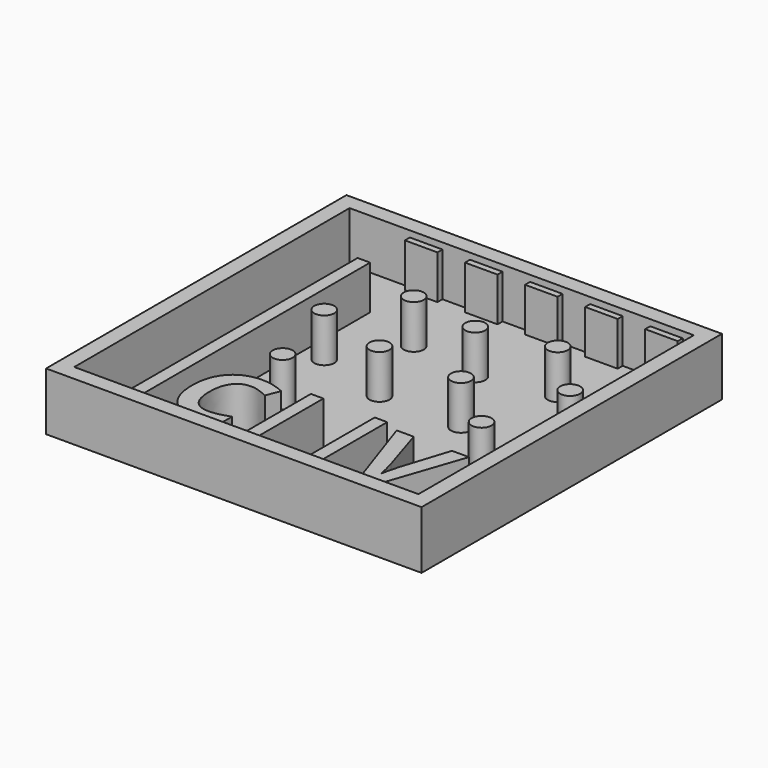
from build123d import *

# Parameters (mm, degrees)
F0_W         = 38.1
F0_H         = 38.1
F1_DEPTH     = 0.79375
F2_W         = 38.1
F2_H         = 38.1
F2_W_2       = 34.925
F2_H_2       = 34.925
F3_DEPTH     = 5.08
F4_R         = 1.27
F5_DEPTH     = 0.396875
F4_W         = 1.27
F4_H         = 29.591
F4_W_2       = 3.302
F4_H_2       = 0.635
F4_TEXT_SIZE = 11.2888888889
F4_R_2       = 1.016
F4_W_3       = 5.207
F4_H_3       = 0.508
F6_DEPTH     = 4.445


# Not quite as in the source:
# - a feature names something its author has since deleted; it is built from what else it names
# - Text() gives the source's letters only with a copy of the font that has no kerning and outlines rounded to 1/6400 em; it was checked with that copy


with BuildPart() as f1:
    # F0 (on Top) → F1 (new body)
    with BuildSketch(Plane.XY):
        with Locations((0, 3.0672513019)):
            Rectangle(F0_W, F0_H)
    extrude(amount=F1_DEPTH)

    # F2 (on face) → F3 (join)
    with BuildSketch(Plane.XY.offset(0.79375)):
        with Locations((0, 3.0672513019)):
            Rectangle(F2_W, F2_H)
        with Locations((0, 3.0672513019)):
            Rectangle(F2_W_2, F2_H_2, mode=Mode.SUBTRACT)
    extrude(amount=F3_DEPTH)

    # F4 (on face) → F5 (cut)
    with BuildSketch(Plane.XY.offset(0.79375)):
        with Locations((-14.9225, -11.5426807876)):
            Circle(F4_R)
        with Locations((3.175, -11.2202486981)):
            Circle(F4_R)
    extrude(amount=-F5_DEPTH, mode=Mode.SUBTRACT)

    # F4 (on face) → F6 (join)
    with BuildSketch(Plane.XY.offset(0.79375)):
        with Locations((-11.7475, 0.4002513019)):
            Rectangle(F4_W, F4_H)
        with Locations((-9.6896662343, 20.2122513019)):
            Rectangle(F4_W_2, F4_H_2)
        with Locations((-3.5936662343, 20.2122513019)):
            Rectangle(F4_W_2, F4_H_2)
        with Locations((2.5023337657, 20.2122513019)):
            Rectangle(F4_W_2, F4_H_2)
        with Locations((8.5983337657, 20.2122513019)):
            Rectangle(F4_W_2, F4_H_2)
        with Locations((14.6943337657, 20.2122513019)):
            Rectangle(F4_W_2, F4_H_2)
        Polygon((5.7785, -13.8872486981), (5.7785, -14.3952486981), (7.0485, -14.3952486981), (7.0485, -5.3331321105), (5.7785, -5.3331321105), align=None)
        with Locations((-9.6321795136, -14.0338847837)):
            Text('C', F4_TEXT_SIZE, font='Open Sans', font_style=FontStyle.BOLD, text_align=(TextAlign.LEFT, TextAlign.BOTTOM))
        with Locations((8.5202609814, -14.0338847837)):
            Text('V', F4_TEXT_SIZE, font='Open Sans', font_style=FontStyle.BOLD, text_align=(TextAlign.LEFT, TextAlign.BOTTOM))
        with Locations((-4.8133307137, 12.8543414176)):
            Circle(F4_R_2)
        with Locations((-8.9067812576, 6.6271641557)):
            Circle(F4_R_2)
        with Locations((14.9268631328, 8.0149960514)):
            Circle(F4_R_2)
        Polygon((-0.6985, -5.3331321105), (-0.6985, -14.3952486981), (0.5715, -14.3952486981), (0.5715, -13.8872486981), (0.5715, -5.3331321105), align=None)
        with Locations((3.175, -14.1412486981)):
            Rectangle(F4_W_3, F4_H_3)
        with Locations((2.2651311961, 11.8151512102)):
            Circle(F4_R_2)
        with Locations((9.4837980851, 13.2500263141)):
            Circle(F4_R_2)
        with Locations((6.7872144282, 4.3443185277)):
            Circle(F4_R_2)
        with Locations((12.8566641361, -0.6274645566)):
            Circle(F4_R_2)
        with Locations((-1.5694284812, 4.4566206634)):
            Circle(F4_R_2)
        with Locations((-6.7170648836, -1.3900776394)):
            Circle(F4_R_2)
    extrude(amount=F6_DEPTH)


solid = f1.part
